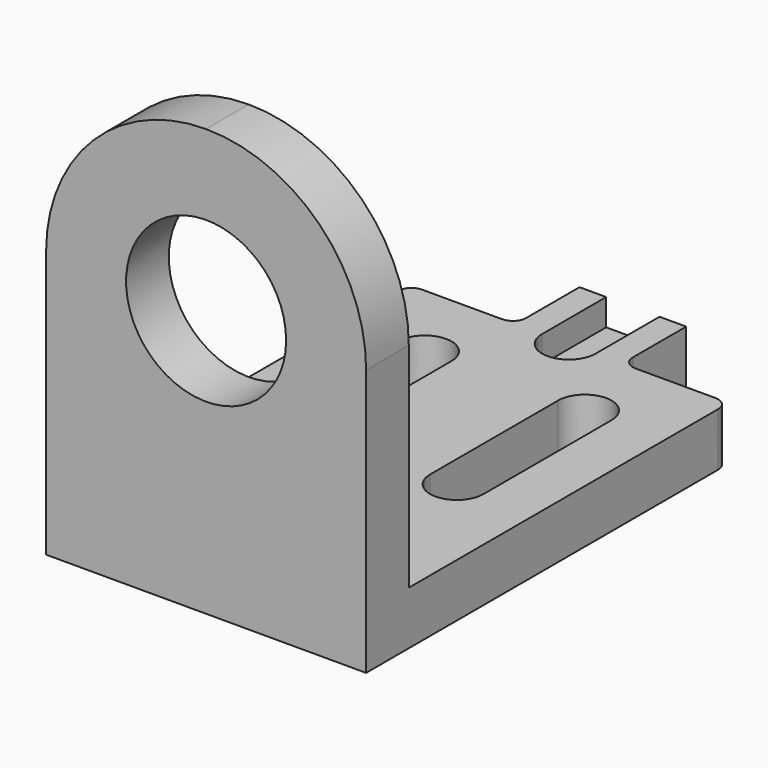
from build123d import *

# Parameters (mm, degrees)
F1_DEPTH = 25.4
F0_W     = 12.7
F0_H     = 31.75
F2_DEPTH = 25.4
F4_DEPTH = 12.7
F6_R     = 38.1
F7_DEPTH = 25.4
F8_DEPTH = 12.7


# Not quite as in the source:
# - a feature names something its author has since deleted; it is built from what else it names


with BuildPart() as f1:
    # F0 (on Top) → F1 (new body)
    with BuildSketch(Plane.XY):
        with BuildLine():
            Line((-76.2, 209.55), (-76.2, 0))
            Line((-76.2, 0), (76.2, 0))
            Line((76.2, 0), (76.2, 209.55))
            ThreePointArc((76.2, 209.55), (74.3401280605, 214.0401280605), (69.85, 215.9))
            Line((69.85, 215.9), (31.75, 215.9))
            ThreePointArc((31.75, 215.9), (27.2598719395, 217.7598719395), (25.4, 222.25))
            Line((25.4, 222.25), (12.7, 222.25))
            Line((12.7, 222.25), (12.7, 215.9))
            ThreePointArc((12.7, 215.9), (0, 203.2), (-12.7, 215.9))
            Line((-12.7, 215.9), (-12.7, 222.25))
            Line((-12.7, 222.25), (-25.4, 222.25))
            ThreePointArc((-25.4, 222.25), (-27.2598719395, 217.7598719395), (-31.75, 215.9))
            Line((-31.75, 215.9), (-69.85, 215.9))
            ThreePointArc((-69.85, 215.9), (-74.3401280605, 214.0401280605), (-76.2, 209.55))
        make_face()
        with BuildLine():
            Line((-50.8, 101.6), (-50.8, 177.8))
            ThreePointArc((-50.8, 177.8), (-38.1, 190.5), (-25.4, 177.8))
            Line((-25.4, 177.8), (-25.4, 101.6))
            ThreePointArc((-25.4, 101.6), (-38.1, 88.9), (-50.8, 101.6))
        make_face(mode=Mode.SUBTRACT)
        with BuildLine():
            Line((25.4, 101.6), (25.4, 177.8))
            ThreePointArc((25.4, 177.8), (38.1, 190.5), (50.8, 177.8))
            Line((50.8, 177.8), (50.8, 101.6))
            ThreePointArc((50.8, 101.6), (38.1, 88.9), (25.4, 101.6))
        make_face(mode=Mode.SUBTRACT)
    extrude(amount=F1_DEPTH)

    # F0 (on Top) → F2 (join)
    with BuildSketch(Plane.XY):
        with Locations((-19.05, 238.125)):
            Rectangle(F0_W, F0_H)
        with Locations((19.05, 238.125)):
            Rectangle(F0_W, F0_H)
    extrude(amount=F2_DEPTH)

    # F3 (on Right) → F4 (join, symmetric)
    with BuildSketch(Plane.YZ):
        Polygon((25.4, 76.2), (25.4, 25.4), (63.5, 25.4), align=None)
    extrude(amount=F4_DEPTH, both=True)

    # F6 (on Front) → F7 (join)
    with BuildSketch(Plane.XZ):
        with BuildLine():
            Line((-76.2, 25.4), (76.2, 25.4))
            Line((76.2, 25.4), (76.2, 127))
            ThreePointArc((76.2, 127), (53.8815367264, 180.8815367264), (0, 203.2))
            ThreePointArc((0, 203.2), (-53.8815367264, 180.8815367264), (-76.2, 127))
            Line((-76.2, 127), (-76.2, 25.4))
        make_face()
        with Locations((0, 127)):
            Circle(F6_R, mode=Mode.SUBTRACT)
    extrude(amount=-F7_DEPTH)

    # F0 (on Top) → F8 (join)
    with BuildSketch(Plane.XY):
        with BuildLine():
            Line((-12.7, 254), (-12.7, 222.25))
            Line((-12.7, 222.25), (-12.7, 215.9))
            ThreePointArc((-12.7, 215.9), (0, 203.2), (12.7, 215.9))
            Line((12.7, 215.9), (12.7, 222.25))
            Line((12.7, 222.25), (12.7, 254))
            Line((12.7, 254), (-12.7, 254))
        make_face()
    extrude(amount=F8_DEPTH)


solid = f1.part
